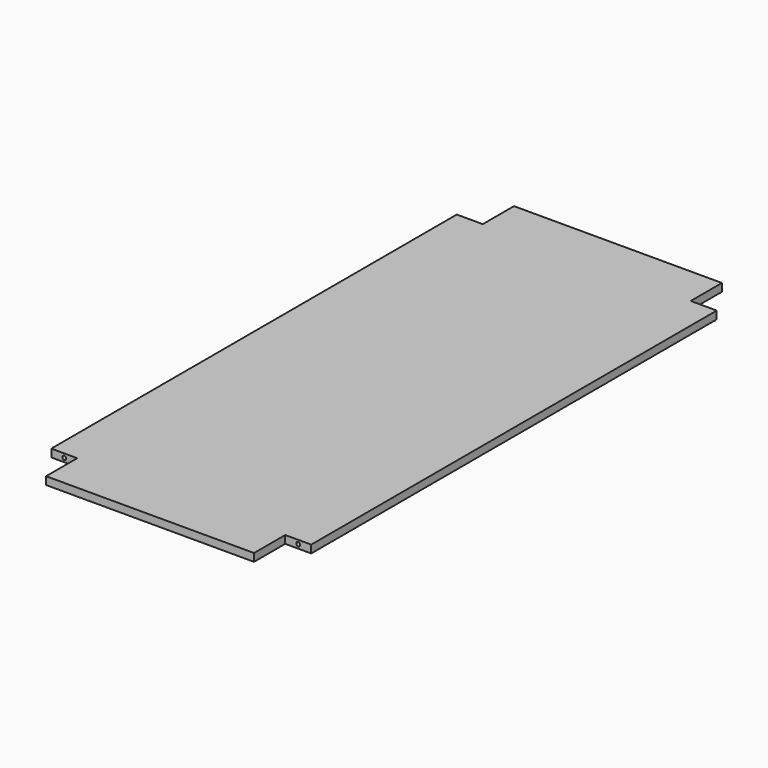
from build123d import *

# Parameters (mm, degrees)
F0_W      = 400
F0_H      = 12
F1_DEPTH  = 450
F2_W      = 40
F2_H      = 60
F3_DEPTH  = 12
F4_W      = 40
F4_H      = 60
F5_DEPTH  = 15
F6_W      = 40
F6_H      = 60
F7_DEPTH  = 15
F8_W      = 40
F8_H      = 60
F9_DEPTH  = 15
F10_R     = 3
F11_DEPTH = 12
F12_R     = 3
F13_DEPTH = 12
F14_R     = 3
F15_DEPTH = 12
F16_R     = 3
F17_DEPTH = 12


with BuildPart() as f1:
    # F0 (on Front) → F1 (new body, symmetric)
    with BuildSketch(Plane.XZ):
        with Locations((200, 6)):
            Rectangle(F0_W, F0_H)
    extrude(amount=F1_DEPTH, both=True)

    # F2 (on face) → F3 (cut)
    with BuildSketch(Plane.XY.offset(12)):
        with Locations((20, 420)):
            Rectangle(F2_W, F2_H)
    extrude(amount=-F3_DEPTH, mode=Mode.SUBTRACT)

    # F4 (on face) → F5 (cut)
    with BuildSketch(Plane.XY.offset(12)):
        with Locations((380, 420)):
            Rectangle(F4_W, F4_H)
    extrude(amount=-F5_DEPTH, mode=Mode.SUBTRACT)

    # F6 (on face) → F7 (cut)
    with BuildSketch(Plane.XY.offset(12)):
        with Locations((380, -420)):
            Rectangle(F6_W, F6_H)
    extrude(amount=-F7_DEPTH, mode=Mode.SUBTRACT)

    # F8 (on face) → F9 (cut)
    with BuildSketch(Plane.XY.offset(12)):
        with Locations((20, -420)):
            Rectangle(F8_W, F8_H)
    extrude(amount=-F9_DEPTH, mode=Mode.SUBTRACT)

    # F10 (on face) → F11 (cut)
    with BuildSketch(Plane.XZ.offset(390)):
        with Locations((20, 6)):
            Circle(F10_R)
    extrude(amount=-F11_DEPTH, mode=Mode.SUBTRACT)

    # F12 (on face) → F13 (cut)
    with BuildSketch(Plane.XZ.offset(390)):
        with Locations((380, 6)):
            Circle(F12_R)
    extrude(amount=-F13_DEPTH, mode=Mode.SUBTRACT)

    # F14 (on face) → F15 (cut)
    with BuildSketch(Plane(origin=(0, 390, 0), x_dir=(-1, 0, 0), z_dir=(0, 1, 0))):
        with Locations((-380, 6)):
            Circle(F14_R)
    extrude(amount=-F15_DEPTH, mode=Mode.SUBTRACT)

    # F16 (on face) → F17 (cut)
    with BuildSketch(Plane(origin=(0, 390, 0), x_dir=(-1, 0, 0), z_dir=(0, 1, 0))):
        with Locations((-20, 6)):
            Circle(F16_R)
    extrude(amount=-F17_DEPTH, mode=Mode.SUBTRACT)


solid = f1.part
